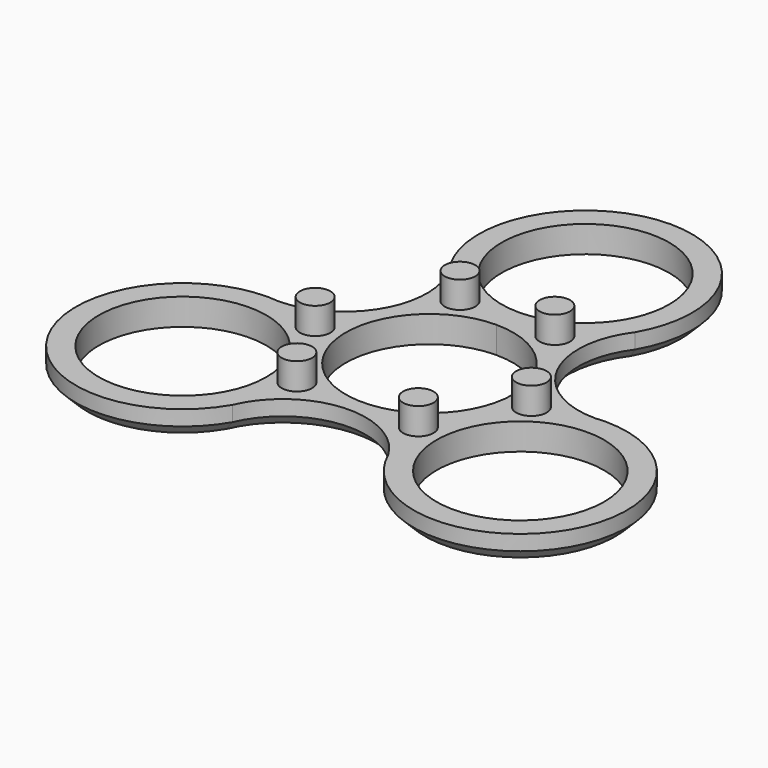
from build123d import *

# Parameters (mm, degrees)
F0_R       = 11
F0_R_2     = 2
F1_DEPTH   = 3.5
F2_DEPTH   = 7
F3_C1_SIZE = 1.5
F3_C2_SIZE = 1.5
F3_C3_SIZE = 1.5
F3_C4_SIZE = 1.5
F3_C5_SIZE = 1.5
F3_C6_SIZE = 1.5


with BuildPart() as f1:
    # F0 (on Top) → F1 (new body)
    with BuildSketch(Plane.XY):
        with BuildLine():
            ThreePointArc((22.164837833, 1.2031249106), (11.390396953, 6.576248747), (12.124355653, 18.5937501788))
            ThreePointArc((12.124355653, 18.5937501788), (0, 39.5937501788), (-12.124355653, 18.5937501788))
            ThreePointArc((-12.124355653, 18.5937501788), (-11.390396953, 6.576248747), (-22.164837833, 1.2031249106))
            ThreePointArc((-22.164837833, 1.2031249106), (-34.2891934859, -19.7968750894), (-10.04048218, -19.7968750894))
            ThreePointArc((-10.04048218, -19.7968750894), (0, -13.152497494), (10.04048218, -19.7968750894))
            ThreePointArc((10.04048218, -19.7968750894), (34.2891934859, -19.7968750894), (22.164837833, 1.2031249106))
        make_face()
        with Locations((-22.164837833, -12.7968750894)):
            Circle(F0_R, mode=Mode.SUBTRACT)
        with Locations((-7.9711980778, -11.7872301109)):
            Circle(F0_R_2, mode=Mode.SUBTRACT)
        with Locations((-14.1936397552, -1.0096449785)):
            Circle(F0_R_2, mode=Mode.SUBTRACT)
        with Locations((7.9711980778, -11.7872301109)):
            Circle(F0_R_2, mode=Mode.SUBTRACT)
        with Locations((22.164837833, -12.7968750894)):
            Circle(F0_R, mode=Mode.SUBTRACT)
        with BuildLine():
            ThreePointArc((0, 11), (7.7781745931, 7.7781745931), (11, 0))
            ThreePointArc((11, 0), (-7.7781745931, -7.7781745931), (0, 11))
        make_face(mode=Mode.SUBTRACT)
        with Locations((14.1936397552, -1.0096449785)):
            Circle(F0_R_2, mode=Mode.SUBTRACT)
        with Locations((-6.2224416774, 12.7968750894)):
            Circle(F0_R_2, mode=Mode.SUBTRACT)
        with Locations((6.2224416774, 12.7968750894)):
            Circle(F0_R_2, mode=Mode.SUBTRACT)
        with BuildLine():
            ThreePointArc((9.5262794416, 20.0937501788), (5.5, 16.0674707372), (0, 14.5937501788))
            ThreePointArc((0, 14.5937501788), (-5.5, 16.0674707372), (-9.5262794416, 20.0937501788))
            ThreePointArc((-9.5262794416, 20.0937501788), (-2.8470094961, 36.218934268), (11, 25.5937501788))
            ThreePointArc((11, 25.5937501788), (10.6251840892, 22.7467406827), (9.5262794416, 20.0937501788))
        make_face(mode=Mode.SUBTRACT)
    extrude(amount=F1_DEPTH)

    # F0 (on Top) → F2 (join)
    with BuildSketch(Plane.XY):
        with Locations((-6.2224416774, 12.7968750894)):
            Circle(F0_R_2)
        with Locations((6.2224416774, 12.7968750894)):
            Circle(F0_R_2)
        with Locations((14.1936397552, -1.0096449785)):
            Circle(F0_R_2)
        with Locations((7.9711980778, -11.7872301109)):
            Circle(F0_R_2)
        with Locations((-7.9711980778, -11.7872301109)):
            Circle(F0_R_2)
        with Locations((-14.1936397552, -1.0096449785)):
            Circle(F0_R_2)
    extrude(amount=F2_DEPTH)

    # F3: chamfer of 1.5 on 6 edges, made by hand

    # F3_c1
    f3_c1_edges = [f1.edges().sort_by_distance(p)[0] for p in [
        (0, -13.152497494, 0),
    ]]
    chamfer(f3_c1_edges, length=F3_C1_SIZE)

    # F3_c2
    f3_c2_edges = [f1.edges().sort_by_distance(p)[0] for p in [
        (11.390396953, 6.576248747, 0),
    ]]
    chamfer(f3_c2_edges, length=F3_C2_SIZE)

    # F3_c3
    f3_c3_edges = [f1.edges().sort_by_distance(p)[0] for p in [
        (-11.390396953, 6.576248747, 0),
    ]]
    chamfer(f3_c3_edges, length=F3_C3_SIZE)

    # F3_c4
    f3_c4_edges = [f1.edges().sort_by_distance(p)[0] for p in [
        (-34.2891934859, -19.7968750894, 0),
    ]]
    chamfer(f3_c4_edges, length=F3_C4_SIZE)

    # F3_c5
    f3_c5_edges = [f1.edges().sort_by_distance(p)[0] for p in [
        (34.2891934859, -19.7968750894, 0),
    ]]
    chamfer(f3_c5_edges, length=F3_C5_SIZE)

    # F3_c6
    f3_c6_edges = [f1.edges().sort_by_distance(p)[0] for p in [
        (0, 39.5937501788, 0),
    ]]
    chamfer(f3_c6_edges, length=F3_C6_SIZE)


solid = f1.part
